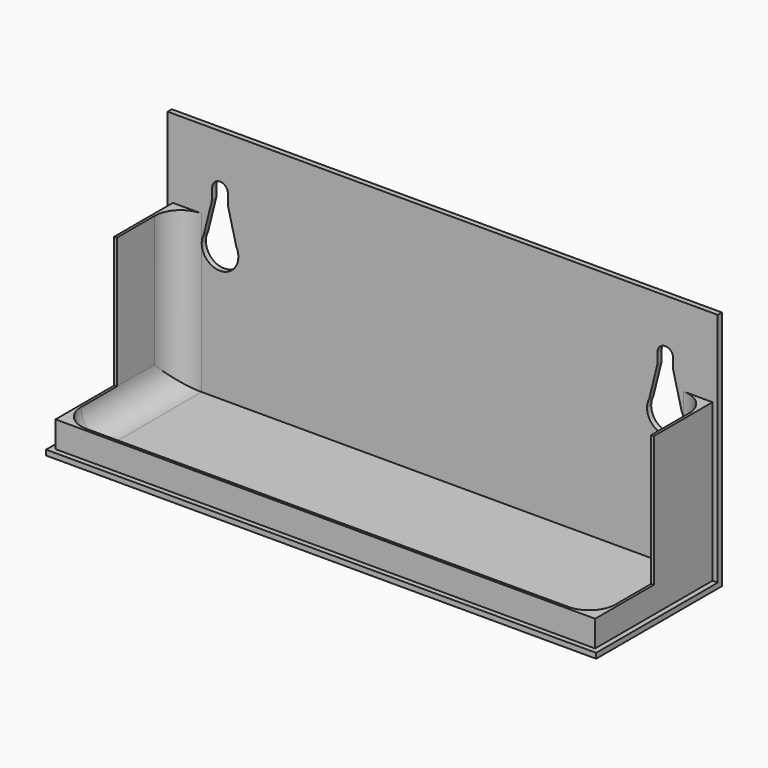
from build123d import *

# Parameters (mm, degrees)
F0_W     = 102
F0_H     = 27.5
F1_DEPTH = 1
F2_DEPTH = 5
F4_DEPTH = 25
F6_DEPTH = 15
F8_DEPTH = 1
F9_R     = 4.99999
F10_R    = 4.99999


# Not quite as in the source:
# - a fillet or chamfer is up to 0.001 mm smaller than in the source, because OpenCascade refuses the exact size
# - a feature names something its author has since deleted; it is built from what else it names


with BuildPart() as f1:
    # F0 (on Top) → F1 (new body)
    with BuildSketch(Plane.XY):
        with Locations((52.5, -14.75)):
            Rectangle(F0_W, F0_H)
        Polygon((1.5, -1), (1, -1), (1, -29), (104, -29), (104, -1), (103.5, -1), (103.5, -28.5), (1.5, -28.5), align=None)
        Polygon((1, -1), (0, -1), (0, -30), (105, -30), (105, -1), (104, -1), (104, -29), (1, -29), align=None)
        Polygon((105, 0), (0, 0), (0, -1), (1, -1), (1.5, -1), (103.5, -1), (104, -1), (105, -1), align=None)
    extrude(amount=-F1_DEPTH)

    # F0 (on Top) → F2 (join)
    with BuildSketch(Plane.XY):
        Polygon((105, 0), (0, 0), (0, -1), (1, -1), (1.5, -1), (103.5, -1), (104, -1), (105, -1), align=None)
        Polygon((1.5, -1), (1, -1), (1, -29), (104, -29), (104, -1), (103.5, -1), (103.5, -28.5), (1.5, -28.5), align=None)
    extrude(amount=F2_DEPTH)

    # F3 (on face) → F4 (join)
    with BuildSketch(Plane.XY.offset(5)):
        Polygon((1, -1), (1, -15), (1.5, -15), (1.5, -1), (103.5, -1), (103.5, -15), (104, -15), (104, -1), (105, -1), (105, 0), (0, 0), (0, -1), align=None)
    extrude(amount=F4_DEPTH)

    # F5 (on face) → F6 (join)
    with BuildSketch(Plane.XY.offset(30)):
        Polygon((1.5, -1), (103.5, -1), (104, -1), (105, -1), (105, 0), (0, 0), (0, -1), (1, -1), align=None)
    extrude(amount=F6_DEPTH)

    # F7 (on face) → F8 (cut, through all)
    with BuildSketch(Plane.XZ.offset(1)):
        with BuildLine():
            Line((13.5, 25), (6.5, 25))
            ThreePointArc((6.5, 25), (10, 21.5), (13.5, 25))
        make_face()
        with BuildLine():
            ThreePointArc((6.9117647059, 26.6470588235), (6.6045012495, 25.8488746876), (6.5, 25))
            Line((6.5, 25), (6.9117647059, 26.6470588235))
        make_face()
        with BuildLine():
            Line((6.9117647059, 26.6470588235), (6.5, 25))
            Line((6.5, 25), (13.5, 25))
            Line((13.5, 25), (13.0882352941, 26.6470588235))
            ThreePointArc((13.0882352941, 26.6470588235), (10, 28.5), (6.9117647059, 26.6470588235))
        make_face()
        with BuildLine():
            Line((13.0882352941, 26.6470588235), (13.5, 25))
            ThreePointArc((13.5, 25), (13.3954987505, 25.8488746876), (13.0882352941, 26.6470588235))
        make_face()
        with BuildLine():
            Line((8.5, 33), (6.9117647059, 26.6470588235))
            ThreePointArc((6.9117647059, 26.6470588235), (10, 28.5), (13.0882352941, 26.6470588235))
            Line((13.0882352941, 26.6470588235), (11.5, 33))
            ThreePointArc((11.5, 33), (10, 31.5), (8.5, 33))
        make_face()
        with BuildLine():
            ThreePointArc((8.8819660113, 34), (8.5987414616, 33.5352331347), (8.5, 33))
            ThreePointArc((8.5, 33), (10, 31.5), (11.5, 33))
            ThreePointArc((11.5, 33), (11.4012585384, 33.5352331347), (11.1180339887, 34))
            ThreePointArc((11.1180339887, 34), (10, 33.5), (8.8819660113, 34))
        make_face()
        with BuildLine():
            Line((8.5, 35), (8.5, 33))
            ThreePointArc((8.5, 33), (8.5987414616, 33.5352331347), (8.8819660113, 34))
            ThreePointArc((8.8819660113, 34), (8.5987414616, 34.4647668653), (8.5, 35))
        make_face()
        with BuildLine():
            ThreePointArc((11.1180339887, 34), (11.4012585384, 33.5352331347), (11.5, 33))
            Line((11.5, 33), (11.5, 35))
            ThreePointArc((11.5, 35), (11.4012585384, 34.4647668653), (11.1180339887, 34))
        make_face()
        with BuildLine():
            ThreePointArc((8.5, 35), (8.5987414616, 34.4647668653), (8.8819660113, 34))
            ThreePointArc((8.8819660113, 34), (10, 34.5), (11.1180339887, 34))
            ThreePointArc((11.1180339887, 34), (11.4012585384, 34.4647668653), (11.5, 35))
            Line((11.5, 35), (8.5, 35))
        make_face()
        with BuildLine():
            ThreePointArc((11.5, 35), (10, 36.5), (8.5, 35))
            Line((8.5, 35), (11.5, 35))
        make_face()
        with BuildLine():
            Line((91.9117647059, 26.6470588235), (91.5, 25))
            ThreePointArc((91.5, 25), (95, 21.5), (98.5, 25))
            Line((98.5, 25), (98.0882352941, 26.6470588235))
            ThreePointArc((98.0882352941, 26.6470588235), (95, 28.5), (91.9117647059, 26.6470588235))
        make_face()
        with BuildLine():
            ThreePointArc((91.9117647059, 26.6470588235), (91.6045012495, 25.8488746876), (91.5, 25))
            Line((91.5, 25), (91.9117647059, 26.6470588235))
        make_face()
        with BuildLine():
            Line((98.0882352941, 26.6470588235), (98.5, 25))
            ThreePointArc((98.5, 25), (98.3954987505, 25.8488746876), (98.0882352941, 26.6470588235))
        make_face()
        with BuildLine():
            Line((93.5, 33), (91.9117647059, 26.6470588235))
            ThreePointArc((91.9117647059, 26.6470588235), (95, 28.5), (98.0882352941, 26.6470588235))
            Line((98.0882352941, 26.6470588235), (96.5, 33))
            ThreePointArc((96.5, 33), (95, 31.5), (93.5, 33))
        make_face()
        with BuildLine():
            ThreePointArc((93.8819660113, 34), (93.5987414616, 33.5352331347), (93.5, 33))
            ThreePointArc((93.5, 33), (95, 31.5), (96.5, 33))
            ThreePointArc((96.5, 33), (96.4012585384, 33.5352331347), (96.1180339887, 34))
            ThreePointArc((96.1180339887, 34), (95, 33.5), (93.8819660113, 34))
        make_face()
        with BuildLine():
            Line((93.5, 35), (93.5, 33))
            ThreePointArc((93.5, 33), (93.5987414616, 33.5352331347), (93.8819660113, 34))
            ThreePointArc((93.8819660113, 34), (93.5987414616, 34.4647668653), (93.5, 35))
        make_face()
        with BuildLine():
            ThreePointArc((96.1180339887, 34), (96.4012585384, 33.5352331347), (96.5, 33))
            Line((96.5, 33), (96.5, 35))
            ThreePointArc((96.5, 35), (96.4012585384, 34.4647668653), (96.1180339887, 34))
        make_face()
        with BuildLine():
            ThreePointArc((93.5, 35), (93.5987414616, 34.4647668653), (93.8819660113, 34))
            ThreePointArc((93.8819660113, 34), (95, 34.5), (96.1180339887, 34))
            ThreePointArc((96.1180339887, 34), (96.4012585384, 34.4647668653), (96.5, 35))
            ThreePointArc((96.5, 35), (95, 36.5), (93.5, 35))
        make_face()
        with BuildLine():
            ThreePointArc((11.1180339887, 34), (10, 34.5), (8.8819660113, 34))
            ThreePointArc((8.8819660113, 34), (10, 33.5), (11.1180339887, 34))
        make_face()
        with BuildLine():
            ThreePointArc((96.1180339887, 34), (95, 34.5), (93.8819660113, 34))
            ThreePointArc((93.8819660113, 34), (95, 33.5), (96.1180339887, 34))
        make_face()
    extrude(amount=-F8_DEPTH, mode=Mode.SUBTRACT)

    # F9 (radius 5 in the source; OpenCascade refuses exactly that, so slightly less here)
    f9_edges = [f1.edges().sort_by_distance(p)[0] for p in [
        (1.5, -14.75, 0),
        (103.5, -14.75, 0),
        (103.5, -1, 15),
        (1.5, -1, 15),
    ]]
    fillet(f9_edges, radius=F9_R)

    # F10 (radius 5 in the source; OpenCascade refuses exactly that, so slightly less here)
    f10_edges = [f1.edges().sort_by_distance(p)[0] for p in [
        (52.5, -28.5, 0),
    ]]
    fillet(f10_edges, radius=F10_R)


solid = f1.part
